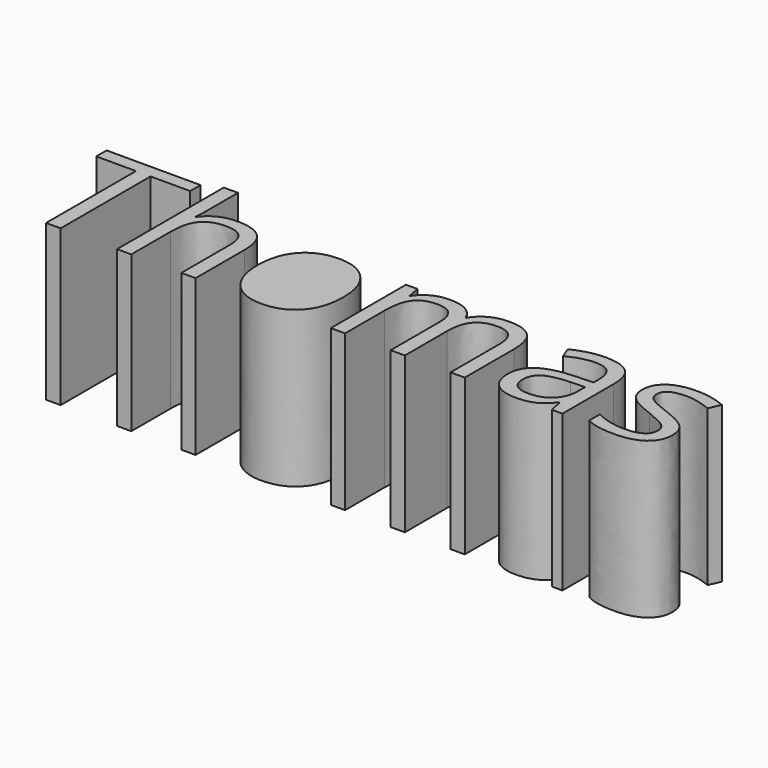
from build123d import *

# Parameters (mm, degrees)
F0_TEXT_SIZE = 45.0977512325
F1_DEPTH     = 40


# Not quite as in the source:
# - Text() gives the source's letters only with a copy of the font that has no kerning and outlines rounded to 1/6400 em; it was checked with that copy


with BuildPart() as f1:
    # F0 (on Top) → F1 (new body)
    with BuildSketch(Plane.XY):
        with Locations((-86.4943750203, 9.0506523848)):
            Text('Thomas', F0_TEXT_SIZE, font='Open Sans', text_align=(TextAlign.LEFT, TextAlign.BOTTOM))
        with BuildLine():
            add(Edge.make_bspline(
                [(-25.714585449, 28.1643477313), (-27.5431583311, 25.8072855771), (-27.5431583311, 21.142486934)],
                knots=[0, 0, 0, 1, 1, 1], degree=2))
            add(Edge.make_bspline(
                [(-27.5431583311, 21.142486934), (-27.5431583311, 16.512920909), (-25.6934458782, 14.0924400421)],
                knots=[0, 0, 0, 1, 1, 1], degree=2))
            add(Edge.make_bspline(
                [(-25.6934458782, 14.0924400421), (-23.8437334253, 11.6719591751), (-20.2570528976, 11.6719591751)],
                knots=[0, 0, 0, 1, 1, 1], degree=2))
            add(Edge.make_bspline(
                [(-20.2570528976, 11.6719591751), (-16.6633258462, 11.6719591751), (-14.8030436079, 14.0818702566)],
                knots=[0, 0, 0, 1, 1, 1], degree=2))
            add(Edge.make_bspline(
                [(-14.8030436079, 14.0818702566), (-12.9427613695, 16.4917813381), (-12.9427613695, 21.142486934)],
                knots=[0, 0, 0, 1, 1, 1], degree=2))
            add(Edge.make_bspline(
                [(-12.9427613695, 21.142486934), (-12.9427613695, 25.7438668644), (-14.8030436079, 28.132638375)],
                knots=[0, 0, 0, 1, 1, 1], degree=2))
            add(Edge.make_bspline(
                [(-14.8030436079, 28.132638375), (-16.6633258462, 30.5214098856), (-20.2993320393, 30.5214098856)],
                knots=[0, 0, 0, 1, 1, 1], degree=2))
            add(Edge.make_bspline(
                [(-20.2993320393, 30.5214098856), (-23.886012567, 30.5214098856), (-25.714585449, 28.1643477313)],
                knots=[0, 0, 0, 1, 1, 1], degree=2))
        make_face()
    extrude(amount=F1_DEPTH)


solid = f1.part
